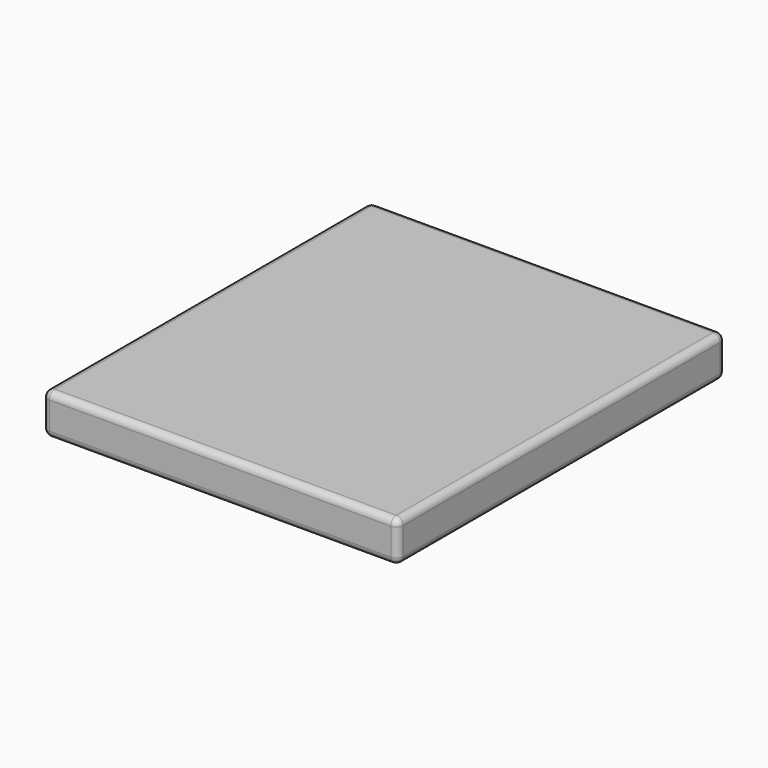
from build123d import *

# Parameters (mm, degrees)
F0_W     = 52
F0_H     = 6
F1_DEPTH = 60
F2_R     = 1


# Not quite as in the source:
# - a feature names something its author has since deleted; it is built from what else it names


with BuildPart() as f1:
    # F0 (on Front) → F1 (new body)
    with BuildSketch(Plane.XZ):
        with Locations((0, 3)):
            Rectangle(F0_W, F0_H)
    extrude(amount=-F1_DEPTH)

    # F2
    f2_edges = [f1.edges().sort_by_distance(p)[0] for p in [
        (0, 60, 6),
        (26, 30, 6),
        (-26, 30, 6),
        (0, 0, 6),
        (26, 60, 3),
        (-26, 60, 3),
        (0, 60, 0),
        (-26, 30, 0),
        (26, 30, 0),
        (0, 0, 0),
        (-26, 0, 3),
        (26, 0, 3),
    ]]
    fillet(f2_edges, radius=F2_R)


solid = f1.part
